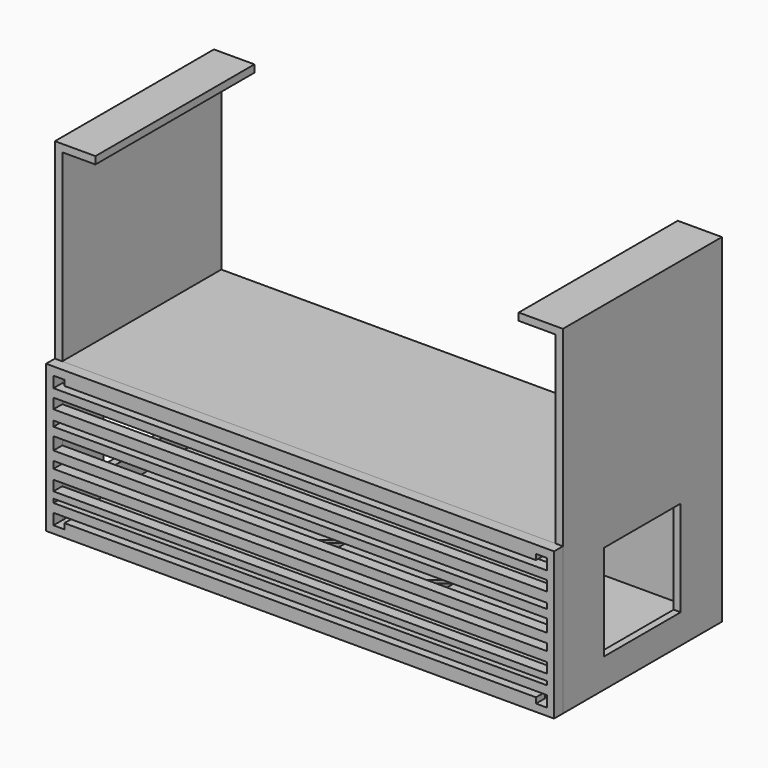
from build123d import *

# Parameters (mm, degrees)
F1_DEPTH  = 540
F2_W      = 130
F2_H      = 130
F3_DEPTH  = 41.5
F5_W      = 130
F5_H      = 260
F6_DEPTH  = 250
F8_DEPTH  = 50
F9_W      = 1380
F9_H      = 400
F9_W_2    = 1340.93075037
F9_H_2    = 10.424464941
F9_H_3    = 27.7985781431
F9_H_4    = 19.1115215421
F9_H_5    = 34.2843079742
F9_H_6    = 14.7630823776
F9_H_7    = 27.7985557914
F11_DEPTH = 30
F10_W     = 1253.9217174053
F10_H     = 5.2477568388
F10_W_2   = 1257.6251924038
F10_H_2   = 7.0648565888
F12_DEPTH = 25
F13_W     = 1340.93075037
F13_H     = 357.9673457496
F14_DEPTH = 20
F16_DEPTH = 50
F18_DEPTH = 25
F20_DEPTH = 25
F21_W     = 270
F21_H     = 30
F22_DEPTH = 11
F23_W     = 50
F23_H     = 50.3848940134
F24_DEPTH = 60


# Not quite as in the source:
# - a feature names something its author has since deleted; it is built from what else it names


with BuildPart() as f1:
    # F0 (on Front) → F1 (new body)
    with BuildSketch(Plane.XZ):
        Polygon((-401.131799221, 210.1073265076), (-401.131799221, 629.3826087959), (-361.131799221, 629.3826087959), (-361.131799221, 649.3826087959), (-421.131799221, 649.3826087959), (-421.131799221, -270.6173912041), (958.868200779, -270.6173912041), (958.868200779, 649.3826087959), (838.868200779, 649.3826087959), (838.868200779, 629.3826087959), (938.868200779, 629.3826087959), (938.868200779, 210.1073265076), (938.868200779, 129.3826087959), (-401.131799221, 129.3826087959), align=None)
        Polygon((938.868200779, -250.6173912041), (-401.131799221, -250.6173912041), (-401.131799221, 107.3499545455), (939.798951149, 107.3499545455), (939.798951149, -250.6173912041), align=None, mode=Mode.SUBTRACT)
    extrude(amount=F1_DEPTH)


with BuildPart() as f3:
    # F2 (on face) → F3 (new body, symmetric)
    with BuildSketch(Plane(origin=(-421.131799221, 0, 0), x_dir=(0, -1, 0), z_dir=(-1, 0, 0))):
        with Locations((205, 3.4951143172)):
            Rectangle(F2_W, F2_H)
        with Locations((335, 3.4951143172)):
            Rectangle(F2_W, F2_H)
        with Locations((335, -126.5048856828)):
            Rectangle(F2_W, F2_H)
        with Locations((205, -126.5048856828)):
            Rectangle(F2_W, F2_H)
    extrude(amount=F3_DEPTH, both=True)


with BuildPart() as f1_1:
    add(f1.part)

    # F4: cut F3
    add(f3.part, mode=Mode.SUBTRACT)


with BuildPart() as f6:
    # F5 (on face) → F6 (new body, symmetric)
    with BuildSketch(Plane.YZ.offset(958.868200779)):
        with Locations((-205, -61.0292432997)):
            Rectangle(F5_W, F5_H)
        with Locations((-335, -61.0292432997)):
            Rectangle(F5_W, F5_H)
    extrude(amount=F6_DEPTH, both=True)


with BuildPart() as f1_2:
    add(f1_1.part)

    # F7: cut F6
    add(f6.part, mode=Mode.SUBTRACT)

    # F8 (add): a face of the model
    f8_faces = [f1_2.faces().sort_by_distance(p)[0] for p in [
        (-361.131799221, -270, 639.3826087959),
    ]]
    extrude(f8_faces, amount=F8_DEPTH)

    # F13 (on face) → F14 (join)
    with BuildSketch(Plane(origin=(0, 0, 0), x_dir=(-1, 0, 0), z_dir=(0, 1, 0))):
        with Locations((-269.333575964, -71.6337183293)):
            Rectangle(F13_W, F13_H)
    extrude(amount=-F14_DEPTH)

    # F15 (on face) → F16 (join)
    with BuildSketch(Plane.XY.offset(-250.6173912041)):
        Polygon((404.333575964, -370), (269.333575964, -370), (134.333575964, -370), (134.333575964, -391.6209638119), (210.3650718927, -391.6209638119), (269.333575964, -391.6209638119), (404.333575964, -391.6209638119), align=None)
    extrude(amount=F16_DEPTH)

    # F17 (on face) → F18 (join)
    with BuildSketch(Plane.YZ.offset(404.333575964)):
        Polygon((-391.6209638119, -200.6173912041), (-391.6209638119, -250.6173912041), (-246.6209638119, -250.6173912041), (-370, -200.6173912041), align=None)
    extrude(amount=F18_DEPTH)

    # F19 (on face) → F20 (join)
    with BuildSketch(Plane(origin=(134.333575964, 0, 0), x_dir=(0, -1, 0), z_dir=(-1, 0, 0))):
        Polygon((246.6209638119, -250.6173912041), (391.6209638119, -250.6173912041), (391.6209638119, -200.6173912041), (370, -200.6173912041), align=None)
    extrude(amount=F20_DEPTH)

    # F21 (on face) → F22 (join)
    with BuildSketch(Plane(origin=(0, -122.0263992007, -301.1099904579), x_dir=(1, 0, 0), z_dir=(0, 0.3755855729, 0.9267877197))):
        with Locations((269.333575964, -252.5624584992)):
            Rectangle(F21_W, F21_H)
    extrude(amount=-F22_DEPTH)


with BuildPart() as f11:
    # F9 (on face) → F11 (new body)
    with BuildSketch(Plane.XZ.offset(540)):
        with Locations((268.868200779, -70.6173912041)):
            Rectangle(F9_W, F9_H)
        Polygon((-371.131799221, -250.6173912041), (-401.131799221, -250.6173912041), (-401.131799221, -220.6173912041), (-371.131799221, -220.6173912041), (909.798951149, -220.6173912041), (939.798951149, -220.6173912041), (939.798951149, -250.6173912041), (909.798951149, -250.6173912041), (909.798951149, -235.6173912041), (-371.131799221, -235.6173912041), align=None, mode=Mode.SUBTRACT)
        with Locations((269.333575964, -191.9789165258)):
            Rectangle(F9_W_2, F9_H_2, mode=Mode.SUBTRACT)
        with Locations((269.333575964, -155.4932966828)):
            Rectangle(F9_W_2, F9_H_3, mode=Mode.SUBTRACT)
        with Locations((269.333575964, -105.9771068394)):
            Rectangle(F9_W_2, F9_H_4, mode=Mode.SUBTRACT)
        with Locations((269.333575964, -54.4915643422)):
            Rectangle(F9_W_2, F9_H_5, mode=Mode.SUBTRACT)
        with Locations((269.333575964, -7.3815411888)):
            Rectangle(F9_W_2, F9_H_6, mode=Mode.SUBTRACT)
        with Locations((269.333575964, 40.834043175)):
            Rectangle(F9_W_2, F9_H_7, mode=Mode.SUBTRACT)
        Polygon((-401.131799221, 77.3499545455), (-401.131799221, 107.3499545455), (-371.131799221, 107.3499545455), (-371.131799221, 92.3499545455), (-364.3079102039, 92.3499545455), (909.798951149, 92.3499545455), (909.798951149, 107.3499545455), (939.798951149, 107.3499545455), (939.798951149, 77.3499545455), (909.798951149, 77.3499545455), (-364.3079102039, 77.3499545455), (-371.131799221, 77.3499545455), align=None, mode=Mode.SUBTRACT)
    extrude(amount=F11_DEPTH)

    # F10 (on face) → F12 (join)
    with BuildSketch(Plane.XZ.offset(540)):
        with Locations((272.5210934877, -246.1882457137)):
            Rectangle(F10_W, F10_H)
        with Locations((270.6693559885, 101.7066277564)):
            Rectangle(F10_W_2, F10_H_2)
    extrude(amount=-F12_DEPTH)


with BuildPart() as f24:
    # F23 (on face) → F24 (new body)
    with BuildSketch(Plane(origin=(0, 0, 0), x_dir=(-1, 0, 0), z_dir=(0, 1, 0))):
        Polygon((-268.868200779, -169.3925857544), (-268.868200779, -219.7774797678), (-218.868200779, -219.7774797678), (-217.6146060228, -219.7774797678), (-217.6146060228, -169.3925857544), align=None)
        with Locations((-293.868200779, -194.5850327611)):
            Rectangle(F23_W, F23_H)
    extrude(amount=-F24_DEPTH)


with BuildPart() as f1_3:
    add(f1_2.part)

    # F25: cut F24
    add(f24.part, mode=Mode.SUBTRACT)


solid = Compound([f11.part, f1_3.part])
